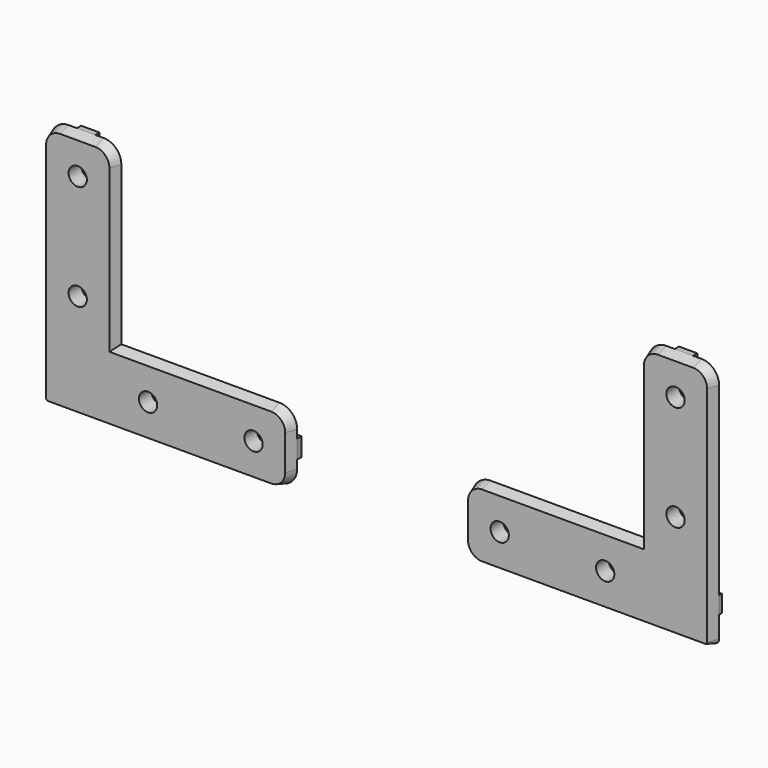
from build123d import *

# Parameters (mm, degrees)
F1_DEPTH = 3
F2_W     = 0.992
F2_H     = 4.86
F3_DEPTH = 20
F4_W     = 5.25
F4_H     = 50
F4_W_2   = 50
F4_H_2   = 5.25
F5_DEPTH = 1.5
F6_R     = 2.6
F7_DEPTH = 4.501
F9_SIZE2 = 0.99999
F9_SIZE  = 2.99999


# Not quite as in the source:
# - a fillet or chamfer is up to 0.001 mm smaller than in the source, because OpenCascade refuses the exact size


with BuildPart() as f1:
    # F0 (on Front) → F1 (new body)
    with BuildSketch(Plane.XZ):
        with BuildLine():
            ThreePointArc((-1.515, 0), (-0.4437332265, 0.4437332265), (0, 1.515))
            Line((0, 1.515), (0, 65))
            ThreePointArc((0, 65), (-1.4644660941, 68.5355339059), (-5, 70))
            Line((-5, 70), (-15, 70))
            ThreePointArc((-15, 70), (-18.5355339059, 68.5355339059), (-20, 65))
            Line((-20, 65), (-20, 20))
            Line((-20, 20), (-65, 20))
            ThreePointArc((-65, 20), (-68.5355339059, 18.5355339059), (-70, 15))
            Line((-70, 15), (-70, 5))
            ThreePointArc((-70, 5), (-68.5355339059, 1.4644660941), (-65, 0))
            Line((-65, 0), (-1.515, 0))
        make_face()
    extrude(amount=F1_DEPTH)

    # F2 (on face) → F3 (join)
    with BuildSketch(Plane.YZ):
        with Locations((0.496, 10)):
            Rectangle(F2_W, F2_H)
    extrude(amount=-F3_DEPTH)

    # F4 (on face) → F5 (join)
    with BuildSketch(Plane(origin=(0, 0, 0), x_dir=(-1, 0, 0), z_dir=(0, 1, 0))):
        with Locations((10, 45)):
            Rectangle(F4_W, F4_H)
        with Locations((45, 10)):
            Rectangle(F4_W_2, F4_H_2)
    extrude(amount=F5_DEPTH)

    # F6 (on face) → F7 (cut, through all)
    with BuildSketch(Plane.XZ.offset(3)):
        with Locations((-10, 60)):
            Circle(F6_R)
        with Locations((-10, 30)):
            Circle(F6_R)
        with Locations((-30, 10)):
            Circle(F6_R)
        with Locations((-60, 10)):
            Circle(F6_R)
    extrude(amount=-F7_DEPTH, mode=Mode.SUBTRACT)

    # F9 (size 3 and 1 in the source; OpenCascade refuses exactly that, so slightly less here)
    f9_edges = [f1.edges().sort_by_distance(p)[0] for p in [
        (-42.5, -3, 20),
    ]]
    f9_side = f1.faces().sort_by_distance((-42.5, -1.5, 20))[0]
    chamfer(f9_edges, length=F9_SIZE, length2=F9_SIZE2, reference=f9_side)


with BuildPart() as f10_1:
    # F10: instance of F1
    add(f1.part.mirror(Plane(origin=(-95, -1.0321782178, 10), x_dir=(0, -1, 0), z_dir=(-1, 0, 0))))


solid = Compound([f1.part, f10_1.part])
